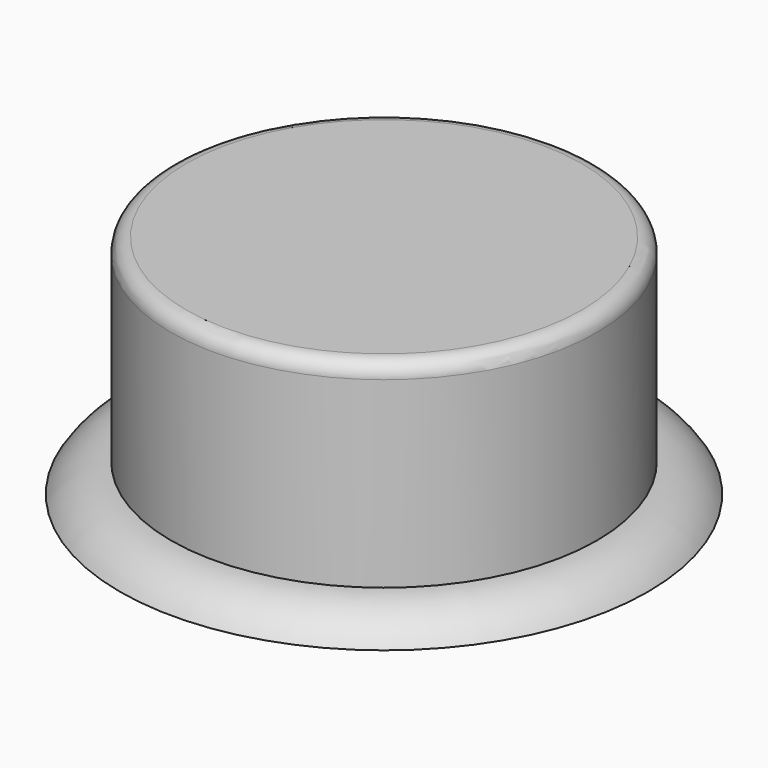
from build123d import *

# Parameters (mm, degrees)
F0_R     = 22.352
F1_DEPTH = 2.413
F3_R     = 18.0284006892
F4_DEPTH = 16.764
F5_R     = 1.27


# Not quite as in the source:
# - a fillet or chamfer that OpenCascade refuses, or shapes differently, is made with other operations: its cross-section is extruded or revolved along the edge and cut away or added


with BuildPart() as f1:
    # F0 (on Top) → F1 (new body)
    with BuildSketch(Plane.XY):
        Circle(F0_R)
    extrude(amount=F1_DEPTH)

    # F2: fillet of radius 5.08 on 1 edges, made by hand

    # F2_s1 → F2_t2 (revolve, cut)
    with BuildSketch(Plane.XZ):
        with BuildLine():
            ThreePointArc((22.352, 0), (20.5040864528, 1.7689192959), (18.0284006892, 2.413))
            Line((18.0284006892, 2.413), (22.352, 2.413))
            Line((22.352, 2.413), (22.352, 0))
        make_face()
    revolve(axis=Axis((0, 0, 2.413), (0, 0, 1)), mode=Mode.SUBTRACT)

    # F3 (on face) → F4 (join)
    with BuildSketch(Plane.XY.offset(2.413)):
        Circle(F3_R)
    extrude(amount=F4_DEPTH)

    # F5
    f5_edges = [f1.edges().sort_by_distance(p)[0] for p in [
        (-18.028401, 0, 19.177),
    ]]
    fillet(f5_edges, radius=F5_R)


solid = f1.part
